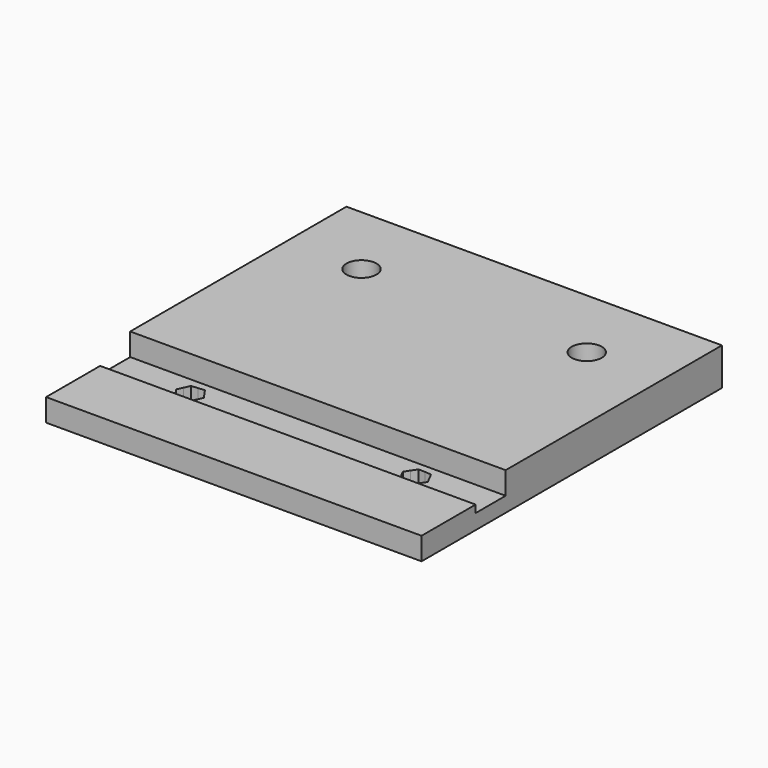
from build123d import *

# Parameters (mm, degrees)
F0_W     = 100
F0_H     = 100
F1_DEPTH = 4
F2_W     = 100
F2_H     = 72
F2_H_2   = 18
F3_DEPTH = 2
F4_W     = 100
F4_H     = 72
F5_DEPTH = 4
F6_R     = 4
F7_DEPTH = 25


with BuildPart() as f1:
    # F0 (on Top) → F1 (new body)
    with BuildSketch(Plane.XY):
        Rectangle(F0_W, F0_H)
    extrude(amount=F1_DEPTH)

    # F2 (on face) → F3 (join)
    with BuildSketch(Plane.XY.offset(4)):
        with Locations((0, 14)):
            Rectangle(F2_W, F2_H)
        with Locations((0, -41)):
            Rectangle(F2_W, F2_H_2)
    extrude(amount=F3_DEPTH)

    # F4 (on face) → F5 (join)
    with BuildSketch(Plane.XY.offset(6)):
        with Locations((0, 14)):
            Rectangle(F4_W, F4_H)
    extrude(amount=F5_DEPTH)

    # F6 (on face) → F7 (cut)
    with BuildSketch(Plane.XY.offset(10)):
        with Locations((30, 30)):
            Circle(F6_R)
        with Locations((-30, 30)):
            Circle(F6_R)
        with BuildLine():
            ThreePointArc((-27.2789726301, -28.3521687498), (-27.0705732549, -27.7357198631), (-27, -27.0888358355))
            ThreePointArc((-27, -27.0888358355), (-27.1396000204, -26.1843404199), (-27.5454079712, -25.3640233899))
            ThreePointArc((-27.5454079712, -25.3640233899), (-28.7366669855, -24.3678085121), (-30.2664349753, -24.1006905237))
            ThreePointArc((-30.2664349753, -24.1006905237), (-31.7248121898, -24.634243627), (-32.721027317, -25.8255028072))
            ThreePointArc((-32.721027317, -25.8255028072), (-32.9881452887, -27.3552710687), (-32.4545920728, -28.8136482183))
            ThreePointArc((-32.4545920728, -28.8136482183), (-31.2633329265, -29.8098631997), (-29.7335647552, -30.0769811231))
            ThreePointArc((-29.7335647552, -30.0769811231), (-28.2751876481, -29.54342793), (-27.2789726301, -28.3521687498))
        make_face()
        with BuildLine():
            ThreePointArc((-27.5454079712, -25.3640233899), (-27.1396000204, -26.1843404199), (-27, -27.0888358355))
            ThreePointArc((-27, -27.0888358355), (-27.0705732549, -27.7357198631), (-27.2789726301, -28.3521687498))
            Line((-27.2789726301, -28.3521687498), (-26.5495870229, -26.7811829673))
            Line((-26.5495870229, -26.7811829673), (-27.5454079712, -25.3640233899))
        make_face()
        with BuildLine():
            ThreePointArc((-30.2664349753, -24.1006905237), (-28.7366669855, -24.3678085121), (-27.5454079712, -25.3640233899))
            Line((-27.5454079712, -25.3640233899), (-28.5412287108, -23.9468641096))
            Line((-28.5412287108, -23.9468641096), (-30.2664349753, -24.1006905237))
        make_face()
        with BuildLine():
            Line((-28.0083583121, -29.9231546931), (-27.2789726301, -28.3521687498))
            ThreePointArc((-27.2789726301, -28.3521687498), (-28.2751876481, -29.54342793), (-29.7335647552, -30.0769811231))
            Line((-29.7335647552, -30.0769811231), (-28.0083583121, -29.9231546931))
        make_face()
        with BuildLine():
            ThreePointArc((-32.721027317, -25.8255028072), (-31.7248121898, -24.634243627), (-30.2664349753, -24.1006905237))
            Line((-30.2664349753, -24.1006905237), (-31.9916416879, -24.2545169778))
            Line((-31.9916416879, -24.2545169778), (-32.721027317, -25.8255028072))
        make_face()
        with BuildLine():
            Line((-31.4587712892, -30.2308075613), (-29.7335647552, -30.0769811231))
            ThreePointArc((-29.7335647552, -30.0769811231), (-31.2633329265, -29.8098631997), (-32.4545920728, -28.8136482183))
            Line((-32.4545920728, -28.8136482183), (-31.4587712892, -30.2308075613))
        make_face()
        with BuildLine():
            ThreePointArc((-32.4545920728, -28.8136482183), (-32.9881452887, -27.3552710687), (-32.721027317, -25.8255028072))
            Line((-32.721027317, -25.8255028072), (-33.4504129771, -27.3964887036))
            Line((-33.4504129771, -27.3964887036), (-32.4545920728, -28.8136482183))
        make_face()
        with BuildLine():
            ThreePointArc((32.5153308801, -28.7239650037), (32.876281683, -27.9416451078), (33, -27.089))
            ThreePointArc((33, -27.089), (32.9172554923, -26.3892712006), (32.6735864049, -25.7281415445))
            ThreePointArc((32.6735864049, -25.7281415445), (31.6349646218, -24.5736688716), (30.1582554561, -24.0931770395))
            ThreePointArc((30.1582554561, -24.0931770395), (28.6391417683, -24.4154134812), (27.4846689431, -25.4540352683))
            ThreePointArc((27.4846689431, -25.4540352683), (27.0041770385, -26.9307445628), (27.3264135035, -28.4498582753))
            ThreePointArc((27.3264135035, -28.4498582753), (28.365035239, -29.6043310379), (29.8417444141, -30.0848229536))
            ThreePointArc((29.8417444141, -30.0848229536), (31.3608580292, -29.7625866218), (32.5153308801, -28.7239650037))
        make_face()
        with BuildLine():
            ThreePointArc((32.6735864049, -25.7281415445), (32.9172554923, -26.3892712006), (33, -27.089))
            ThreePointArc((33, -27.089), (32.876281683, -27.9416451078), (32.5153308801, -28.7239650037))
            Line((32.5153308801, -28.7239650037), (33.4592783853, -27.2717376616))
            Line((33.4592783853, -27.2717376616), (32.6735864049, -25.7281415445))
        make_face()
        with BuildLine():
            ThreePointArc((30.1582554561, -24.0931770395), (31.6349646218, -24.5736688716), (32.6735864049, -25.7281415445))
            Line((32.6735864049, -25.7281415445), (31.8878946499, -24.1845458704))
            Line((31.8878946499, -24.1845458704), (30.1582554561, -24.0931770395))
        make_face()
        with BuildLine():
            Line((31.5713837355, -30.1761917913), (32.5153308801, -28.7239650037))
            ThreePointArc((32.5153308801, -28.7239650037), (31.3608580292, -29.7625866218), (29.8417444141, -30.0848229536))
            Line((29.8417444141, -30.0848229536), (31.5713837355, -30.1761917913))
        make_face()
        with BuildLine():
            ThreePointArc((27.4846689431, -25.4540352683), (28.6391417683, -24.4154134812), (30.1582554561, -24.0931770395))
            Line((30.1582554561, -24.0931770395), (28.4286162645, -24.0018082087))
            Line((28.4286162645, -24.0018082087), (27.4846689431, -25.4540352683))
        make_face()
        with BuildLine():
            Line((28.1121053501, -29.9934541296), (29.8417444141, -30.0848229536))
            ThreePointArc((29.8417444141, -30.0848229536), (28.365035239, -29.6043310379), (27.3264135035, -28.4498582753))
            Line((27.3264135035, -28.4498582753), (28.1121053501, -29.9934541296))
        make_face()
        with BuildLine():
            ThreePointArc((27.3264135035, -28.4498582753), (27.0041770385, -26.9307445628), (27.4846689431, -25.4540352683))
            Line((27.4846689431, -25.4540352683), (26.5407216147, -26.9062623384))
            Line((26.5407216147, -26.9062623384), (27.3264135035, -28.4498582753))
        make_face()
    extrude(amount=-F7_DEPTH, mode=Mode.SUBTRACT)


solid = f1.part
